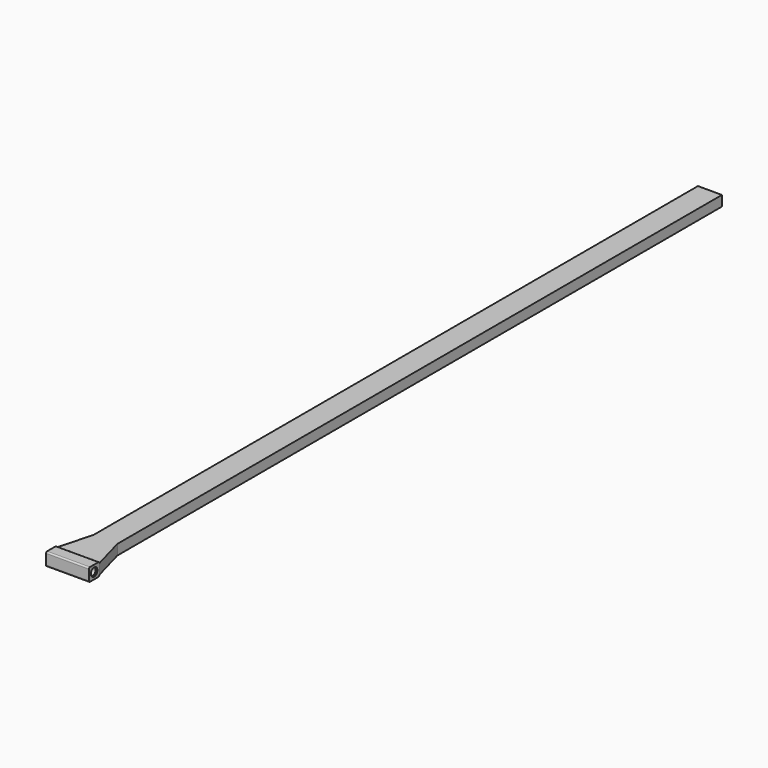
from build123d import *

# Parameters (mm, degrees)
F0_R     = 60
F0_R_2   = 53.033
F1_DEPTH = 312.5
F2_R     = 52.5
F3_DEPTH = 625.001
F2_R_2   = 60
F4_DEPTH = 20
F6_DEPTH = 75
F8_W     = 335
F8_H     = 135
F9_DEPTH = 11530.001


# Not quite as in the source:
# - a pattern or mirror of a feature is missing from the dataset's text; its kind, count and spacing are read off the source's solid


with BuildPart() as f1:
    # F0 (on Right) → F1 (new body, symmetric)
    with BuildSketch(Plane.YZ):
        with BuildLine():
            Line((75, 95), (-75, 95))
            ThreePointArc((-75, 95), (-89.1421356237, 89.1421356237), (-95, 75))
            Line((-95, 75), (-95, -75))
            ThreePointArc((-95, -75), (-89.1421356237, -89.1421356237), (-75, -95))
            Line((-75, -95), (75, -95))
            ThreePointArc((75, -95), (89.1421356237, -89.1421356237), (95, -75))
            Line((95, -75), (95, 75))
            ThreePointArc((95, 75), (89.1421356237, 89.1421356237), (75, 95))
        make_face()
        Circle(F0_R, mode=Mode.SUBTRACT)
        Circle(F0_R)
        Circle(F0_R_2, mode=Mode.SUBTRACT)
        Circle(F0_R_2)
    extrude(amount=F1_DEPTH, both=True)

    # F2 (on face) → F3 (cut, through all)
    with BuildSketch(Plane.YZ.offset(312.5)):
        Circle(F2_R)
    extrude(amount=-F3_DEPTH, mode=Mode.SUBTRACT)

    # F2 (on face) → F4 (cut)
    with BuildSketch(Plane.YZ.offset(312.5)):
        Circle(F2_R_2)
        Circle(F2_R, mode=Mode.SUBTRACT)
    f4 = extrude(amount=-F4_DEPTH, mode=Mode.SUBTRACT)

    # F4_copies: F4 across plane
    add(f4.mirror(Plane(origin=(0, 0, 0), x_dir=(0, 0, -1), z_dir=(-1, 0, 0))), mode=Mode.SUBTRACT)

    # F5 (on Top) → F6 (join, symmetric)
    with BuildSketch(Plane.XY):
        Polygon((-312.5, 95), (312.5, 95), (175, 595), (175, 11620), (0, 11620), (-175, 11620), (-175, 595), align=None)
    extrude(amount=F6_DEPTH, both=True)

    # F8 (on offset) → F9 (cut, through all)
    with BuildSketch(Plane.XZ.offset(-90)):
        Rectangle(F8_W, F8_H)
    extrude(amount=-F9_DEPTH, mode=Mode.SUBTRACT)


solid = f1.part
